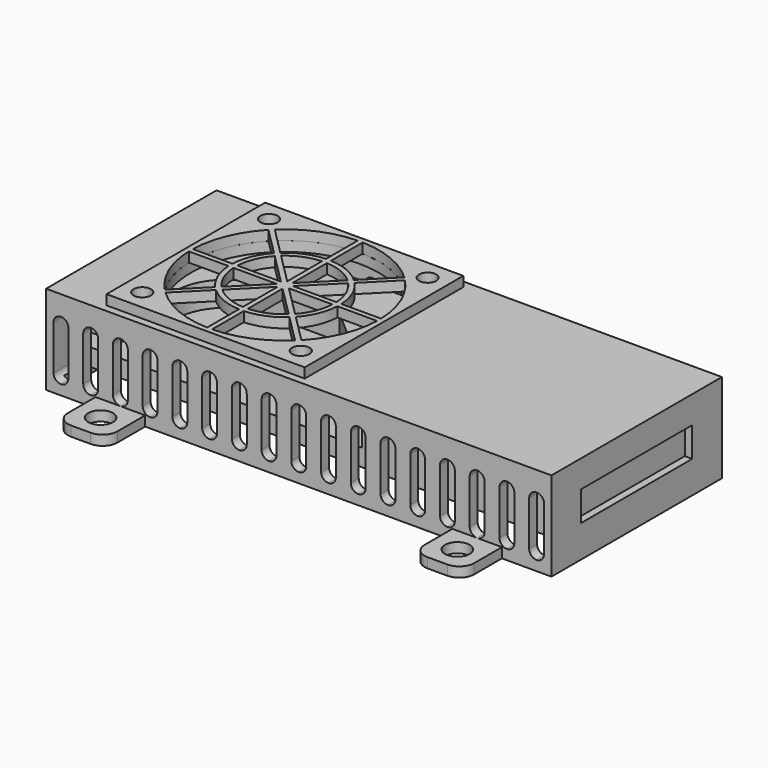
from build123d import *

# Parameters (mm, degrees)
F1_W      = 96
F1_H      = 37
F2_DEPTH  = 8.5
F4_DEPTH  = 5
F5_W      = 27
F5_H      = 27
F6_DEPTH  = 2
F7_W      = 102
F7_H      = 43
F7_W_2    = 98
F7_H_2    = 39
F8_DEPTH  = 16
F10_DEPTH = 43.001
F11_W     = 28
F11_H     = 6
F12_DEPTH = 1.5
F13_W     = 20
F13_H     = 10
F14_DEPTH = 1.8829660113
F15_W     = 102
F15_H     = 43
F15_R     = 1.75
F15_R_2   = 19
F16_DEPTH = 2
F17_R     = 2.5
F18_DEPTH = 2
F19_W     = 40
F19_H     = 40
F19_R     = 1.75
F20_DEPTH = 2


with BuildPart() as f2:
    # F1 (on Top) → F2 (new body)
    with BuildSketch(Plane.XY):
        Rectangle(F1_W, F1_H)
    extrude(amount=F2_DEPTH)

    # F3 (on face) → F4 (cut)
    with BuildSketch(Plane.XY.offset(8.5)):
        with BuildLine():
            Line((-44, -14.5), (-48, -14.5))
            Line((-48, -14.5), (-48, -18.5))
            Line((-48, -18.5), (10.4, -18.5))
            Line((10.4, -18.5), (10.4, -2.8))
            Line((10.4, -2.8), (-3.1, -2.8))
            Line((-3.1, -2.8), (-15, 7.5))
            Line((-15, 7.5), (-30, 7.5))
            ThreePointArc((-30, 7.5), (-37.0710678119, 4.5710678119), (-40, -2.5))
            Line((-40, -2.5), (-40, -10.5))
            ThreePointArc((-40, -10.5), (-41.1715728753, -13.3284271247), (-44, -14.5))
        make_face()
    extrude(amount=-F4_DEPTH, mode=Mode.SUBTRACT)

    # F5 (on face) → F6 (join)
    with BuildSketch(Plane(origin=(0, 0, 0), x_dir=(1, 0, 0), z_dir=(0, 0, -1))):
        with Locations((18.5, 0)):
            Rectangle(F5_W, F5_H)
    extrude(amount=F6_DEPTH)


with BuildPart() as f8:
    # F7 (on offset) → F8 (new body)
    with BuildSketch(Plane.XY.offset(-5)):
        Rectangle(F7_W, F7_H)
        Rectangle(F7_W_2, F7_H_2, mode=Mode.SUBTRACT)
    extrude(amount=F8_DEPTH)

    # F9 (on face) → F10 (cut, through all)
    with BuildSketch(Plane.XZ.offset(21.5)):
        with BuildLine():
            Line((1.5, -1.5), (1.5, 7.5))
            ThreePointArc((1.5, 7.5), (1.0606601718, 8.5606601718), (0, 9))
            ThreePointArc((0, 9), (-1.0606601718, 8.5606601718), (-1.5, 7.5))
            Line((-1.5, 7.5), (-1.5, -1.5))
            ThreePointArc((-1.5, -1.5), (-1.0606601718, -2.5606601718), (0, -3))
            ThreePointArc((0, -3), (1.0606601718, -2.5606601718), (1.5, -1.5))
        make_face()
        with BuildLine():
            ThreePointArc((6, 9), (4.9393398282, 8.5606601718), (4.5, 7.5))
            Line((4.5, 7.5), (4.5, -1.5))
            ThreePointArc((4.5, -1.5), (4.9393398282, -2.5606601718), (6, -3))
            ThreePointArc((6, -3), (7.0606601718, -2.5606601718), (7.5, -1.5))
            Line((7.5, -1.5), (7.5, 7.5))
            ThreePointArc((7.5, 7.5), (7.0606601718, 8.5606601718), (6, 9))
        make_face()
        with BuildLine():
            ThreePointArc((12, 9), (10.9393398282, 8.5606601718), (10.5, 7.5))
            Line((10.5, 7.5), (10.5, -1.5))
            ThreePointArc((10.5, -1.5), (10.9393398282, -2.5606601718), (12, -3))
            ThreePointArc((12, -3), (13.0606601718, -2.5606601718), (13.5, -1.5))
            Line((13.5, -1.5), (13.5, 7.5))
            ThreePointArc((13.5, 7.5), (13.0606601718, 8.5606601718), (12, 9))
        make_face()
        with BuildLine():
            ThreePointArc((18, 9), (16.9393398282, 8.5606601718), (16.5, 7.5))
            Line((16.5, 7.5), (16.5, -1.5))
            ThreePointArc((16.5, -1.5), (16.9393398282, -2.5606601718), (18, -3))
            ThreePointArc((18, -3), (19.0606601718, -2.5606601718), (19.5, -1.5))
            Line((19.5, -1.5), (19.5, 7.5))
            ThreePointArc((19.5, 7.5), (19.0606601718, 8.5606601718), (18, 9))
        make_face()
        with BuildLine():
            ThreePointArc((24, 9), (22.9393398282, 8.5606601718), (22.5, 7.5))
            Line((22.5, 7.5), (22.5, -1.5))
            ThreePointArc((22.5, -1.5), (22.9393398282, -2.5606601718), (24, -3))
            ThreePointArc((24, -3), (25.0606601718, -2.5606601718), (25.5, -1.5))
            Line((25.5, -1.5), (25.5, 7.5))
            ThreePointArc((25.5, 7.5), (25.0606601718, 8.5606601718), (24, 9))
        make_face()
        with BuildLine():
            ThreePointArc((30, 9), (28.9393398282, 8.5606601718), (28.5, 7.5))
            Line((28.5, 7.5), (28.5, -1.5))
            ThreePointArc((28.5, -1.5), (28.9393398282, -2.5606601718), (30, -3))
            ThreePointArc((30, -3), (31.0606601718, -2.5606601718), (31.5, -1.5))
            Line((31.5, -1.5), (31.5, 7.5))
            ThreePointArc((31.5, 7.5), (31.0606601718, 8.5606601718), (30, 9))
        make_face()
        with BuildLine():
            ThreePointArc((36, 9), (34.9393398282, 8.5606601718), (34.5, 7.5))
            Line((34.5, 7.5), (34.5, -1.5))
            ThreePointArc((34.5, -1.5), (34.9393398282, -2.5606601718), (36, -3))
            ThreePointArc((36, -3), (37.0606601718, -2.5606601718), (37.5, -1.5))
            Line((37.5, -1.5), (37.5, 7.5))
            ThreePointArc((37.5, 7.5), (37.0606601718, 8.5606601718), (36, 9))
        make_face()
        with BuildLine():
            ThreePointArc((42, 9), (40.9393398282, 8.5606601718), (40.5, 7.5))
            Line((40.5, 7.5), (40.5, -1.5))
            ThreePointArc((40.5, -1.5), (40.9393398282, -2.5606601718), (42, -3))
            ThreePointArc((42, -3), (43.0606601718, -2.5606601718), (43.5, -1.5))
            Line((43.5, -1.5), (43.5, 7.5))
            ThreePointArc((43.5, 7.5), (43.0606601718, 8.5606601718), (42, 9))
        make_face()
        with BuildLine():
            ThreePointArc((48, 9), (46.9393398282, 8.5606601718), (46.5, 7.5))
            Line((46.5, 7.5), (46.5, -1.5))
            ThreePointArc((46.5, -1.5), (46.9393398282, -2.5606601718), (48, -3))
            ThreePointArc((48, -3), (49.0606601718, -2.5606601718), (49.5, -1.5))
            Line((49.5, -1.5), (49.5, 7.5))
            ThreePointArc((49.5, 7.5), (49.0606601718, 8.5606601718), (48, 9))
        make_face()
        with BuildLine():
            ThreePointArc((-4.5, 7.5), (-4.9393398282, 8.5606601718), (-6, 9))
            ThreePointArc((-6, 9), (-7.0606601718, 8.5606601718), (-7.5, 7.5))
            Line((-7.5, 7.5), (-7.5, -1.5))
            ThreePointArc((-7.5, -1.5), (-7.0606601718, -2.5606601718), (-6, -3))
            ThreePointArc((-6, -3), (-4.9393398282, -2.5606601718), (-4.5, -1.5))
            Line((-4.5, -1.5), (-4.5, 7.5))
        make_face()
        with BuildLine():
            ThreePointArc((-48, -3), (-46.9393398282, -2.5606601718), (-46.5, -1.5))
            Line((-46.5, -1.5), (-46.5, 7.5))
            ThreePointArc((-46.5, 7.5), (-46.9393398282, 8.5606601718), (-48, 9))
            ThreePointArc((-48, 9), (-49.0606601718, 8.5606601718), (-49.5, 7.5))
            Line((-49.5, 7.5), (-49.5, -1.5))
            ThreePointArc((-49.5, -1.5), (-49.0606601718, -2.5606601718), (-48, -3))
        make_face()
        with BuildLine():
            ThreePointArc((-40.5, 7.5), (-40.9393398282, 8.5606601718), (-42, 9))
            ThreePointArc((-42, 9), (-43.0606601718, 8.5606601718), (-43.5, 7.5))
            Line((-43.5, 7.5), (-43.5, -1.5))
            ThreePointArc((-43.5, -1.5), (-43.0606601718, -2.5606601718), (-42, -3))
            ThreePointArc((-42, -3), (-40.9393398282, -2.5606601718), (-40.5, -1.5))
            Line((-40.5, -1.5), (-40.5, 7.5))
        make_face()
        with BuildLine():
            ThreePointArc((-34.5, 7.5), (-34.9393398282, 8.5606601718), (-36, 9))
            ThreePointArc((-36, 9), (-37.0606601718, 8.5606601718), (-37.5, 7.5))
            Line((-37.5, 7.5), (-37.5, -1.5))
            ThreePointArc((-37.5, -1.5), (-37.0606601718, -2.5606601718), (-36, -3))
            ThreePointArc((-36, -3), (-34.9393398282, -2.5606601718), (-34.5, -1.5))
            Line((-34.5, -1.5), (-34.5, 7.5))
        make_face()
        with BuildLine():
            ThreePointArc((-12, -3), (-10.9393398282, -2.5606601718), (-10.5, -1.5))
            Line((-10.5, -1.5), (-10.5, 7.5))
            ThreePointArc((-10.5, 7.5), (-10.9393398282, 8.5606601718), (-12, 9))
            ThreePointArc((-12, 9), (-13.0606601718, 8.5606601718), (-13.5, 7.5))
            Line((-13.5, 7.5), (-13.5, -1.5))
            ThreePointArc((-13.5, -1.5), (-13.0606601718, -2.5606601718), (-12, -3))
        make_face()
        with BuildLine():
            ThreePointArc((-18, -3), (-16.9393398282, -2.5606601718), (-16.5, -1.5))
            Line((-16.5, -1.5), (-16.5, 7.5))
            ThreePointArc((-16.5, 7.5), (-16.9393398282, 8.5606601718), (-18, 9))
            ThreePointArc((-18, 9), (-19.0606601718, 8.5606601718), (-19.5, 7.5))
            Line((-19.5, 7.5), (-19.5, -1.5))
            ThreePointArc((-19.5, -1.5), (-19.0606601718, -2.5606601718), (-18, -3))
        make_face()
        with BuildLine():
            ThreePointArc((-24, -3), (-22.9393398282, -2.5606601718), (-22.5, -1.5))
            Line((-22.5, -1.5), (-22.5, 7.5))
            ThreePointArc((-22.5, 7.5), (-22.9393398282, 8.5606601718), (-24, 9))
            ThreePointArc((-24, 9), (-25.0606601718, 8.5606601718), (-25.5, 7.5))
            Line((-25.5, 7.5), (-25.5, -1.5))
            ThreePointArc((-25.5, -1.5), (-25.0606601718, -2.5606601718), (-24, -3))
        make_face()
        with BuildLine():
            ThreePointArc((-30, -3), (-28.9393398282, -2.5606601718), (-28.5, -1.5))
            Line((-28.5, -1.5), (-28.5, 7.5))
            ThreePointArc((-28.5, 7.5), (-28.9393398282, 8.5606601718), (-30, 9))
            ThreePointArc((-30, 9), (-31.0606601718, 8.5606601718), (-31.5, 7.5))
            Line((-31.5, 7.5), (-31.5, -1.5))
            ThreePointArc((-31.5, -1.5), (-31.0606601718, -2.5606601718), (-30, -3))
        make_face()
    extrude(amount=-F10_DEPTH, mode=Mode.SUBTRACT)

    # F11 (on face) → F12 (cut, through all)
    with BuildSketch(Plane.YZ.offset(51)):
        with Locations((0, 4.5)):
            Rectangle(F11_W, F11_H)
    extrude(amount=-F12_DEPTH, mode=Mode.SUBTRACT)

    # F13 (on face) → F14 (cut, through all)
    with BuildSketch(Plane(origin=(-51, 0, 0), x_dir=(0, -1, 0), z_dir=(-1, 0, 0))):
        with Locations((0, 3.5)):
            Rectangle(F13_W, F13_H)
    extrude(amount=-F14_DEPTH, mode=Mode.SUBTRACT)

    # F15 (on face) → F16 (join)
    with BuildSketch(Plane.XY.offset(11)):
        Rectangle(F15_W, F15_H)
        with Locations((-36, -16)):
            Circle(F15_R, mode=Mode.SUBTRACT)
        with Locations((-4, -16)):
            Circle(F15_R, mode=Mode.SUBTRACT)
        with Locations((-20, 0)):
            Circle(F15_R_2, mode=Mode.SUBTRACT)
        with Locations((-36, 16)):
            Circle(F15_R, mode=Mode.SUBTRACT)
        with Locations((-4, 16)):
            Circle(F15_R, mode=Mode.SUBTRACT)
    extrude(amount=F16_DEPTH)

    # F17 (on offset) → F18 (join)
    with BuildSketch(Plane.XY.offset(-5)):
        with BuildLine():
            Line((-31, -21.5), (-41, -21.5))
            Line((-41, -21.5), (-41, -28.5))
            ThreePointArc((-41, -28.5), (-40.1213203436, -30.6213203436), (-38, -31.5))
            Line((-38, -31.5), (-34, -31.5))
            ThreePointArc((-34, -31.5), (-31.8786796564, -30.6213203436), (-31, -28.5))
            Line((-31, -28.5), (-31, -21.5))
        make_face()
        with Locations((-36, -26.5)):
            Circle(F17_R, mode=Mode.SUBTRACT)
        with BuildLine():
            ThreePointArc((31, -28.5), (31.8786796564, -30.6213203436), (34, -31.5))
            Line((34, -31.5), (38, -31.5))
            ThreePointArc((38, -31.5), (40.1213203436, -30.6213203436), (41, -28.5))
            Line((41, -28.5), (41, -21.5))
            Line((41, -21.5), (31, -21.5))
            Line((31, -21.5), (31, -28.5))
        make_face()
        with Locations((36, -26.5)):
            Circle(F17_R, mode=Mode.SUBTRACT)
        with BuildLine():
            Line((38, 31.5), (34, 31.5))
            ThreePointArc((34, 31.5), (31.8786796564, 30.6213203436), (31, 28.5))
            Line((31, 28.5), (31, 21.5))
            Line((31, 21.5), (41, 21.5))
            Line((41, 21.5), (41, 28.5))
            ThreePointArc((41, 28.5), (40.1213203436, 30.6213203436), (38, 31.5))
        make_face()
        with Locations((36, 26.5)):
            Circle(F17_R, mode=Mode.SUBTRACT)
        with BuildLine():
            ThreePointArc((-38, 31.5), (-40.1213203436, 30.6213203436), (-41, 28.5))
            Line((-41, 28.5), (-41, 21.5))
            Line((-41, 21.5), (-31, 21.5))
            Line((-31, 21.5), (-31, 28.5))
            ThreePointArc((-31, 28.5), (-31.8786796564, 30.6213203436), (-34, 31.5))
            Line((-34, 31.5), (-38, 31.5))
        make_face()
        with Locations((-36, 26.5)):
            Circle(F17_R, mode=Mode.SUBTRACT)
    extrude(amount=F18_DEPTH)


with BuildPart() as f20:
    # F19 (on face) → F20 (new body)
    with BuildSketch(Plane.XY.offset(13)):
        with Locations((-20, 0)):
            Rectangle(F19_W, F19_H)
        with Locations((-36, -16)):
            Circle(F19_R, mode=Mode.SUBTRACT)
        with BuildLine():
            ThreePointArc((-20.5, -18.9934199132), (-27.2709852149, -17.5537111177), (-33.076822628, -13.7839294092))
            Line((-33.076822628, -13.7839294092), (-27.4165817434, -8.1236885246))
            ThreePointArc((-27.4165817434, -8.1236885246), (-24.209517756, -10.1626748576), (-20.5, -10.9886304879))
            Line((-20.5, -10.9886304879), (-20.5, -18.9934199132))
        make_face(mode=Mode.SUBTRACT)
        with BuildLine():
            ThreePointArc((-33.7839294092, -13.076822628), (-37.5537111177, -7.2709852149), (-38.9934199132, -0.5))
            Line((-38.9934199132, -0.5), (-30.9886304879, -0.5))
            ThreePointArc((-30.9886304879, -0.5), (-30.1626748576, -4.209517756), (-28.1236885246, -7.4165817434))
            Line((-28.1236885246, -7.4165817434), (-33.7839294092, -13.076822628))
        make_face(mode=Mode.SUBTRACT)
        with BuildLine():
            Line((-26.7086700553, -7.4157768365), (-20.5, -1.2071067812))
            Line((-20.5, -1.2071067812), (-20.5, -9.9874921777))
            ThreePointArc((-20.5, -9.9874921777), (-23.8268343237, -9.2387953251), (-26.7086700553, -7.4157768365))
        make_face(mode=Mode.SUBTRACT)
        with BuildLine():
            ThreePointArc((-27.4157768365, -6.7086700553), (-29.2387953251, -3.8268343237), (-29.9874921777, -0.5))
            Line((-29.9874921777, -0.5), (-21.2071067812, -0.5))
            Line((-21.2071067812, -0.5), (-27.4157768365, -6.7086700553))
        make_face(mode=Mode.SUBTRACT)
        with BuildLine():
            ThreePointArc((-6.923177372, -13.7839294092), (-12.7290147851, -17.5537111177), (-19.5, -18.9934199132))
            Line((-19.5, -18.9934199132), (-19.5, -10.9886304879))
            ThreePointArc((-19.5, -10.9886304879), (-15.790482244, -10.1626748576), (-12.5834182566, -8.1236885246))
            Line((-12.5834182566, -8.1236885246), (-6.923177372, -13.7839294092))
        make_face(mode=Mode.SUBTRACT)
        with Locations((-4, -16)):
            Circle(F19_R, mode=Mode.SUBTRACT)
        with BuildLine():
            Line((-19.5, -9.9874921777), (-19.5, -1.2071067812))
            Line((-19.5, -1.2071067812), (-13.2913299447, -7.4157768365))
            ThreePointArc((-13.2913299447, -7.4157768365), (-16.1731656763, -9.2387953251), (-19.5, -9.9874921777))
        make_face(mode=Mode.SUBTRACT)
        with BuildLine():
            ThreePointArc((-10.0125078223, -0.5), (-10.7612046749, -3.8268343237), (-12.5842231635, -6.7086700553))
            Line((-12.5842231635, -6.7086700553), (-18.7928932188, -0.5))
            Line((-18.7928932188, -0.5), (-10.0125078223, -0.5))
        make_face(mode=Mode.SUBTRACT)
        with BuildLine():
            Line((-6.2160705908, -13.076822628), (-11.8763114754, -7.4165817434))
            ThreePointArc((-11.8763114754, -7.4165817434), (-9.8373251424, -4.209517756), (-9.0113695121, -0.5))
            Line((-9.0113695121, -0.5), (-1.0065800868, -0.5))
            ThreePointArc((-1.0065800868, -0.5), (-2.4462888823, -7.2709852149), (-6.2160705908, -13.076822628))
        make_face(mode=Mode.SUBTRACT)
        with BuildLine():
            ThreePointArc((-38.9934199132, 0.5), (-37.5537111177, 7.2709852149), (-33.7839294092, 13.076822628))
            Line((-33.7839294092, 13.076822628), (-28.1236885246, 7.4165817434))
            ThreePointArc((-28.1236885246, 7.4165817434), (-30.1626748576, 4.209517756), (-30.9886304879, 0.5))
            Line((-30.9886304879, 0.5), (-38.9934199132, 0.5))
        make_face(mode=Mode.SUBTRACT)
        with BuildLine():
            Line((-27.4157768365, 6.7086700553), (-21.2071067812, 0.5))
            Line((-21.2071067812, 0.5), (-29.9874921777, 0.5))
            ThreePointArc((-29.9874921777, 0.5), (-29.2387953251, 3.8268343237), (-27.4157768365, 6.7086700553))
        make_face(mode=Mode.SUBTRACT)
        with BuildLine():
            Line((-20.5, 9.9874921777), (-20.5, 1.2071067812))
            Line((-20.5, 1.2071067812), (-26.7086700553, 7.4157768365))
            ThreePointArc((-26.7086700553, 7.4157768365), (-23.8268343237, 9.2387953251), (-20.5, 9.9874921777))
        make_face(mode=Mode.SUBTRACT)
        with Locations((-36, 16)):
            Circle(F19_R, mode=Mode.SUBTRACT)
        with BuildLine():
            ThreePointArc((-33.076822628, 13.7839294092), (-27.2709852149, 17.5537111177), (-20.5, 18.9934199132))
            Line((-20.5, 18.9934199132), (-20.5, 10.9886304879))
            ThreePointArc((-20.5, 10.9886304879), (-24.209517756, 10.1626748576), (-27.4165817434, 8.1236885246))
            Line((-27.4165817434, 8.1236885246), (-33.076822628, 13.7839294092))
        make_face(mode=Mode.SUBTRACT)
        with BuildLine():
            Line((-10.0125078223, 0.5), (-18.7928932188, 0.5))
            Line((-18.7928932188, 0.5), (-12.5842231635, 6.7086700553))
            ThreePointArc((-12.5842231635, 6.7086700553), (-10.7612046749, 3.8268343237), (-10.0125078223, 0.5))
        make_face(mode=Mode.SUBTRACT)
        with BuildLine():
            ThreePointArc((-19.5, 9.9874921777), (-16.1731656763, 9.2387953251), (-13.2913299447, 7.4157768365))
            Line((-13.2913299447, 7.4157768365), (-19.5, 1.2071067812))
            Line((-19.5, 1.2071067812), (-19.5, 9.9874921777))
        make_face(mode=Mode.SUBTRACT)
        with BuildLine():
            Line((-1.0065800868, 0.5), (-9.0113695121, 0.5))
            ThreePointArc((-9.0113695121, 0.5), (-9.8373251424, 4.209517756), (-11.8763114754, 7.4165817434))
            Line((-11.8763114754, 7.4165817434), (-6.2160705908, 13.076822628))
            ThreePointArc((-6.2160705908, 13.076822628), (-2.4462888823, 7.2709852149), (-1.0065800868, 0.5))
        make_face(mode=Mode.SUBTRACT)
        with BuildLine():
            ThreePointArc((-19.5, 18.9934199132), (-12.7290147851, 17.5537111177), (-6.923177372, 13.7839294092))
            Line((-6.923177372, 13.7839294092), (-12.5834182566, 8.1236885246))
            ThreePointArc((-12.5834182566, 8.1236885246), (-15.790482244, 10.1626748576), (-19.5, 10.9886304879))
            Line((-19.5, 10.9886304879), (-19.5, 18.9934199132))
        make_face(mode=Mode.SUBTRACT)
        with Locations((-4, 16)):
            Circle(F19_R, mode=Mode.SUBTRACT)
    extrude(amount=F20_DEPTH)


solid = Compound([f2.part, f8.part, f20.part])
